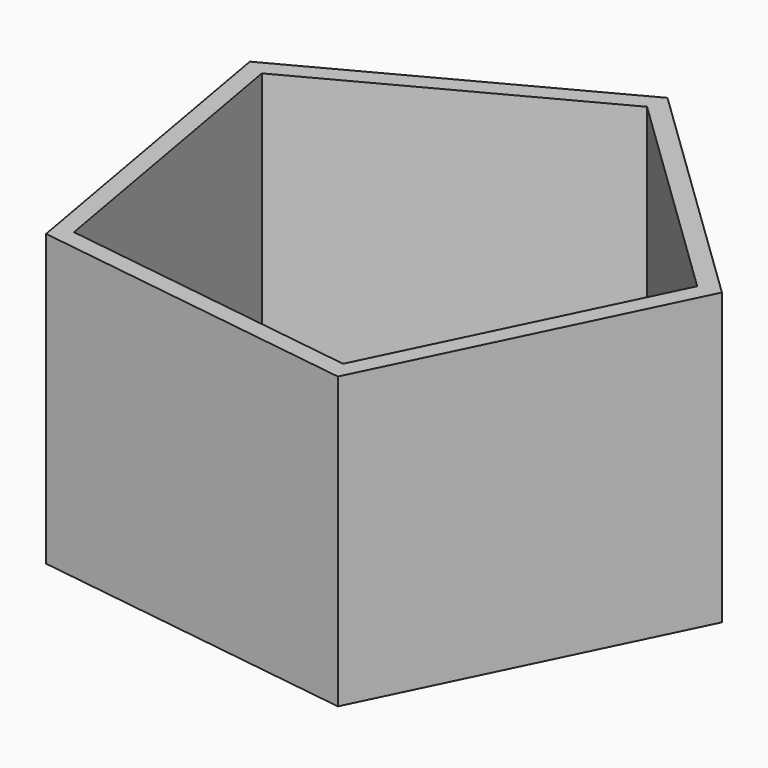
from build123d import *

# Parameters (mm, degrees)
F1_DEPTH = 177.8
F2_T     = -10.8857142857


# Not quite as in the source:
# - a length typed as a fraction of an inch, garbled in the dataset ("3 / 203.2 mm" for 3/8 in), is restored


with BuildPart() as f1:
    # F0 (on Top) → F1 (new body)
    with BuildSketch(Plane.XY):
        Polygon((24.0005461687, 171.1778961441), (-155.3832769332, 75.7227547983), (-120.0326925967, -124.378659957), (81.1989931472, -152.5929941269), (170.216430214, 30.0710031415), align=None)
    extrude(amount=F1_DEPTH)

    # F2
    f2_openings = [f1.faces().sort_by_distance(p)[0] for p in [
        (0, 0, 177.8),
    ]]
    offset(amount=F2_T, openings=f2_openings)


solid = f1.part
